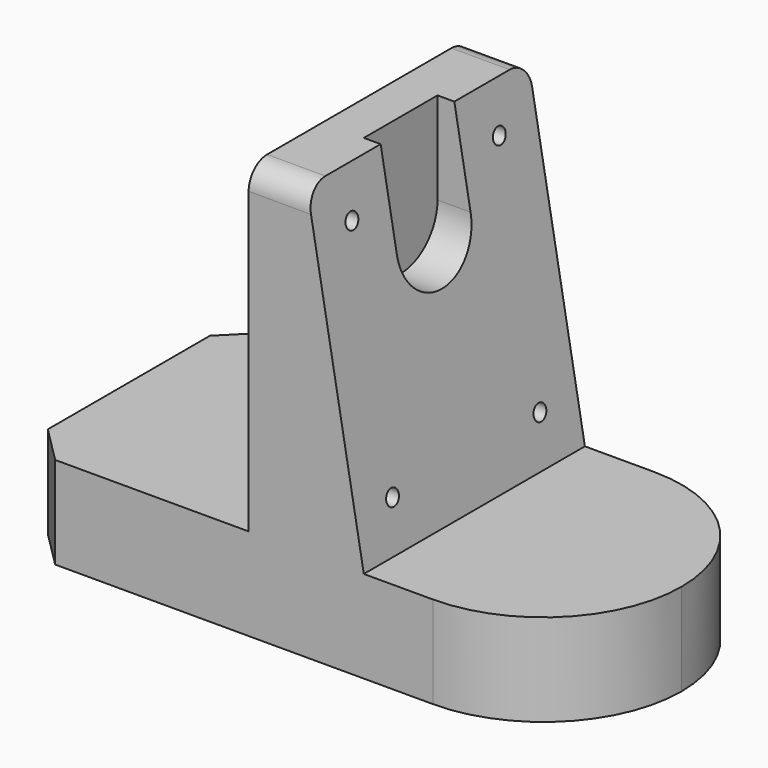
from build123d import *

# Parameters (mm, degrees)
F1_DEPTH       = 30
F2_R           = 29.99999
F4_D           = 3.4
F4_CBORE_D     = 7
F4_CBORE_DEPTH = 2
F5_SIZE        = 8
F10_DEPTH      = 16
F11_DEPTH      = 60.001
F12_R          = 5


# Not quite as in the source:
# - a fillet or chamfer is up to 0.001 mm smaller than in the source, because OpenCascade refuses the exact size


with BuildPart() as f1:
    # F0 (on Front) → F1 (new body, symmetric)
    with BuildSketch(Plane.XZ):
        Polygon((0, 20), (0, 0), (120, 0), (120, 20), (75, 20), (75, 90), (50, 90), (50, 20), align=None)
    extrude(amount=F1_DEPTH, both=True)

    # F2 (radius 30 in the source; OpenCascade refuses exactly that, so slightly less here)
    f2_edges = [f1.edges().sort_by_distance(p)[0] for p in [
        (120, -30, 10),
        (120, 30, 10),
    ]]
    fillet(f2_edges, radius=F2_R)

    # F4 (through all)
    with Locations(Plane(origin=(50, 0, 0), x_dir=(0, -1, 0), z_dir=(-1, 0, 0))):
        with Locations((-20, 80), (-20, 30), (20, 30), (20, 80)):
            CounterBoreHole(F4_D / 2, F4_CBORE_D / 2, F4_CBORE_DEPTH)

    # F5
    f5_edges = [f1.edges().sort_by_distance(p)[0] for p in [
        (0, 30, 10),
        (0, -30, 10),
    ]]
    chamfer(f5_edges, length=F5_SIZE)

    # F7 (on face) → F10 (cut, through all)
    with BuildSketch(Plane.YZ.offset(75)):
        with BuildLine():
            ThreePointArc((-10, 70), (0, 80), (10, 70))
            Line((10, 70), (10, 90))
            Line((10, 90), (-10, 90))
            Line((-10, 90), (-10, 70))
        make_face()
        with BuildLine():
            ThreePointArc((-10, 70), (0, 60), (10, 70))
            ThreePointArc((10, 70), (0, 80), (-10, 70))
        make_face()
    extrude(amount=-F10_DEPTH, mode=Mode.SUBTRACT)

    # F6 (on face) → F11 (cut, through all)
    with BuildSketch(Plane.XZ.offset(30)):
        Polygon((62.6571113504, 90), (75, 20), (75, 90), align=None)
    extrude(amount=-F11_DEPTH, mode=Mode.SUBTRACT)

    # F12
    f12_edges = [f1.edges().sort_by_distance(p)[0] for p in [
        (56.328556, -30, 90),
        (56.328556, 30, 90),
    ]]
    fillet(f12_edges, radius=F12_R)


solid = f1.part
